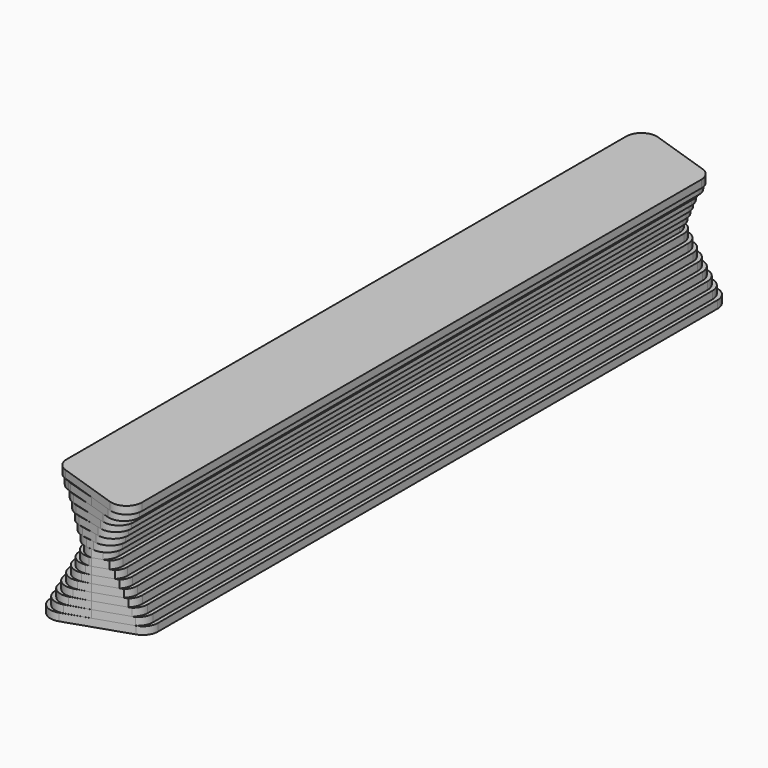
from build123d import *

# Parameters (mm, degrees)
F1_DEPTH  = 6.35
F3_DEPTH  = 6.35
F5_DEPTH  = 6.35
F7_DEPTH  = 6.35
F9_DEPTH  = 6.35
F11_DEPTH = 6.35
F13_DEPTH = 6.35
F15_DEPTH = 6.35
F17_DEPTH = 6.35
F19_DEPTH = 6.35
F21_DEPTH = 6.35
F23_DEPTH = 6.35
F25_DEPTH = 6.35
F27_DEPTH = 6.35
F29_DEPTH = 6.35
F31_DEPTH = 6.35
F33_DEPTH = 6.35


# Not quite as in the source:
# - a feature of the source that left no trace in its solid (it failed there, or was rolled back) is left out


with BuildPart() as f1:
    # F0 (on Top) → F1 (new body)
    with BuildSketch(Plane.XY):
        with BuildLine():
            Line((-38.1, 295.6463579053), (-38.1, 0))
            Line((-38.1, 0), (-38.1, -287.1796912386))
            ThreePointArc((-38.1, -287.1796912386), (-32.8258206152, -297.4824669904), (-21.3839073716, -299.2279691239))
            Line((-21.3839073716, -299.2279691239), (29.4160926284, -282.2946357905))
            ThreePointArc((29.4160926284, -282.2946357905), (35.7027757517, -277.6721785205), (38.1, -270.2463579053))
            Line((38.1, -270.2463579053), (38.1, 0))
            Line((38.1, 0), (38.1, 312.5796912386))
            ThreePointArc((38.1, 312.5796912386), (32.8258206152, 322.8824669904), (21.3839073716, 324.6279691239))
            Line((21.3839073716, 324.6279691239), (-29.4160926284, 307.6946357905))
            ThreePointArc((-29.4160926284, 307.6946357905), (-35.7027757517, 303.0721785205), (-38.1, 295.6463579053))
        make_face()
    extrude(amount=F1_DEPTH)


with BuildPart() as f3:
    # F2 (on face) → F3 (new body)
    with BuildSketch(Plane.XY.offset(6.35)):
        with BuildLine():
            Line((-34.925, 297.1010332697), (-34.925, 0))
            Line((-34.925, 0), (-34.925, -285.8442150878))
            ThreePointArc((-34.925, -285.8442150878), (-29.7212084455, -296.0958909967), (-18.3743135526, -297.946372494))
            Line((-18.3743135526, -297.946372494), (0, -292.1))
            Line((0, -292.1), (29.0322054134, -282.4225981955))
            ThreePointArc((29.0322054134, -282.4225981955), (33.3547239128, -277.8181605059), (34.925, -271.7010332697))
            Line((34.925, -271.7010332697), (34.925, 0))
            Line((34.925, 0), (34.925, 311.2442150878))
            ThreePointArc((34.925, 311.2442150878), (29.7212084455, 321.4958909967), (18.3743135526, 323.346372494))
            Line((18.3743135526, 323.346372494), (0, 317.5))
            Line((0, 317.5), (-29.0322054134, 307.8225981955))
            ThreePointArc((-29.0322054134, 307.8225981955), (-33.3547239128, 303.2181605059), (-34.925, 297.1010332697))
        make_face()
    extrude(amount=F3_DEPTH)


with BuildPart() as f5:
    # F4 (on face) → F5 (new body)
    with BuildSketch(Plane.XY.offset(12.7)):
        with BuildLine():
            Line((-31.75, 298.5258107337), (-31.75, 0))
            Line((-31.75, 0), (-31.75, -284.5558107337))
            ThreePointArc((-31.75, -284.5558107337), (-26.6310177264, -294.744930923), (-15.4006818533, -296.720204556))
            Line((-15.4006818533, -296.720204556), (0, -292.1))
            Line((0, -292.1), (26.8461437511, -283.1512854163))
            ThreePointArc((26.8461437511, -283.1512854163), (30.4583527654, -278.7060873559), (31.75, -273.1258107337))
            Line((31.75, -273.1258107337), (31.75, 0))
            Line((31.75, 0), (31.75, 309.9558107337))
            ThreePointArc((31.75, 309.9558107337), (26.6310177264, 320.144930923), (15.4006818533, 322.120204556))
            Line((15.4006818533, 322.120204556), (0, 317.5))
            Line((0, 317.5), (-26.8461437511, 308.5512854163))
            ThreePointArc((-26.8461437511, 308.5512854163), (-30.4583527654, 304.1060873559), (-31.75, 298.5258107337))
        make_face()
    extrude(amount=F5_DEPTH)


with BuildPart() as f7:
    # F6 (on face) → F7 (new body)
    with BuildSketch(Plane.XY.offset(19.05)):
        with BuildLine():
            Line((-28.575, 299.9094122505), (-28.575, 0))
            Line((-28.575, 0), (-28.575, -283.3288566949))
            ThreePointArc((-28.575, -283.3288566949), (-23.5601064147, -293.4396993598), (-12.4759229299, -295.5655341472))
            Line((-12.4759229299, -295.5655341472), (0, -292.1))
            Line((0, -292.1), (24.3225747643, -283.9924750786))
            ThreePointArc((24.3225747643, -283.9924750786), (27.4632310882, -279.7058437421), (28.575, -274.5094122505))
            Line((28.575, -274.5094122505), (28.575, 0))
            Line((28.575, 0), (28.575, 308.7288566949))
            ThreePointArc((28.575, 308.7288566949), (23.5601064147, 318.8396993598), (12.4759229299, 320.9655341472))
            Line((12.4759229299, 320.9655341472), (0, 317.5))
            Line((0, 317.5), (-24.3225747643, 309.3924750786))
            ThreePointArc((-24.3225747643, 309.3924750786), (-27.4632310882, 305.1058437421), (-28.575, 299.9094122505))
        make_face()
    extrude(amount=F7_DEPTH)


with BuildPart() as f9:
    # F8 (on face) → F9 (new body)
    with BuildSketch(Plane.XY.offset(25.4)):
        with BuildLine():
            Line((-25.4, 301.2341396387), (-25.4, 0))
            Line((-25.4, 0), (-25.4, -282.1841396387))
            ThreePointArc((-25.4, -282.1841396387), (-20.5157350594, -292.1943487015), (-9.619797562, -294.5049493905))
            Line((-9.619797562, -294.5049493905), (0, -292.1))
            Line((0, -292.1), (21.5906498503, -284.9031167166))
            ThreePointArc((21.5906498503, -284.9031167166), (24.4089976748, -280.7524089939), (25.4, -275.8341396387))
            Line((25.4, -275.8341396387), (25.4, 0))
            Line((25.4, 0), (25.4, 307.5841396387))
            ThreePointArc((25.4, 307.5841396387), (20.5157350594, 317.5943487015), (9.619797562, 319.9049493905))
            Line((9.619797562, 319.9049493905), (0, 317.5))
            Line((0, 317.5), (-21.5906498503, 310.3031167166))
            ThreePointArc((-21.5906498503, 310.3031167166), (-24.4089976748, 306.1524089939), (-25.4, 301.2341396387))
        make_face()
    extrude(amount=F9_DEPTH)


with BuildPart() as f11:
    # F10 (on face) → F11 (new body)
    with BuildSketch(Plane.XY.offset(31.75)):
        with BuildLine():
            Line((-22.225, 302.470619464), (-22.225, 0))
            Line((-22.225, 0), (-22.225, -281.1527623212))
            ThreePointArc((-22.225, -281.1527623212), (-17.509204822, -291.0291216383), (-6.8639805731, -293.57085298))
            Line((-6.8639805731, -293.57085298), (0, -292.1))
            Line((0, -292.1), (18.679051767, -285.873649411))
            ThreePointArc((18.679051767, -285.873649411), (21.3052049524, -281.8158034731), (22.225, -277.070619464))
            Line((22.225, -277.070619464), (22.225, 0))
            Line((22.225, 0), (22.225, 306.5527623212))
            ThreePointArc((22.225, 306.5527623212), (17.509204822, 316.4291216383), (6.8639805731, 318.97085298))
            Line((6.8639805731, 318.97085298), (0, 317.5))
            Line((0, 317.5), (-18.679051767, 311.273649411))
            ThreePointArc((-18.679051767, 311.273649411), (-21.3052049524, 307.2158034731), (-22.225, 302.470619464))
        make_face()
    extrude(amount=F11_DEPTH)


with BuildPart() as f13:
    # F12 (on face) → F13 (new body)
    with BuildSketch(Plane.XY.offset(38.1)):
        with BuildLine():
            Line((-19.05, 303.5664859775), (-19.05, 0))
            Line((-19.05, 0), (-19.05, -280.2831526442))
            ThreePointArc((-19.05, -280.2831526442), (-14.5589611809, -289.9735064216), (-4.2621328612, -292.8103554769))
            Line((-4.2621328612, -292.8103554769), (0, -292.1))
            Line((0, -292.1), (15.5567073259, -286.9144308914))
            ThreePointArc((15.5567073259, -286.9144308914), (18.1443881367, -282.8763064073), (19.05, -278.1664859775))
            Line((19.05, -278.1664859775), (19.05, 0))
            Line((19.05, 0), (19.05, 305.6831526442))
            ThreePointArc((19.05, 305.6831526442), (14.5589611809, 315.3735064216), (4.2621328612, 318.2103554769))
            Line((4.2621328612, 318.2103554769), (0, 317.5))
            Line((0, 317.5), (-15.5567073259, 312.3144308914))
            ThreePointArc((-15.5567073259, 312.3144308914), (-18.1443881367, 308.2763064073), (-19.05, 303.5664859775))
        make_face()
    extrude(amount=F13_DEPTH)


with BuildPart() as f15:
    # F14 (on face) → F15 (new body)
    with BuildSketch(Plane.XY.offset(44.45)):
        with BuildLine():
            Line((-15.875, 304.4191579612), (-15.875, 0))
            Line((-15.875, 0), (-15.875, -279.6541579612))
            ThreePointArc((-15.875, -279.6541579612), (-11.6967675737, -289.0706051373), (-1.9113027684, -292.2911302768))
            Line((-1.9113027684, -292.2911302768), (0, -292.1))
            Line((0, -292.1), (12.0810941165, -288.0729686278))
            ThreePointArc((12.0810941165, -288.0729686278), (14.8881847778, -283.9274471091), (15.875, -279.0191579612))
            Line((15.875, -279.0191579612), (15.875, 0))
            Line((15.875, 0), (15.875, 305.0541579612))
            ThreePointArc((15.875, 305.0541579612), (11.6967675737, 314.4706051373), (1.9113027684, 317.6911302768))
            Line((1.9113027684, 317.6911302768), (0, 317.5))
            Line((0, 317.5), (-12.0810941165, 313.4729686278))
            ThreePointArc((-12.0810941165, 313.4729686278), (-14.8881847778, 309.3274471091), (-15.875, 304.4191579612))
        make_face()
    extrude(amount=F15_DEPTH)


with BuildPart() as f17:
    # F16 (on face) → F17 (new body)
    with BuildSketch(Plane.XY.offset(50.8)):
        with BuildLine():
            Line((-12.7, 304.8), (-12.7, 0))
            Line((-12.7, 0), (-12.7, -279.4))
            ThreePointArc((-12.7, -279.4), (-8.9802561211, -288.3802561211), (0, -292.1))
            Line((0, -292.1), (7.62, -289.56))
            ThreePointArc((7.62, -289.56), (11.3592253257, -285.0796126628), (12.7, -279.4))
            Line((12.7, -279.4), (12.7, 0))
            Line((12.7, 0), (12.7, 304.8))
            ThreePointArc((12.7, 304.8), (8.9802561211, 313.7802561211), (0, 317.5))
            Line((0, 317.5), (-7.62, 314.96))
            ThreePointArc((-7.62, 314.96), (-11.3592253257, 310.4796126628), (-12.7, 304.8))
        make_face()
    extrude(amount=F17_DEPTH)


with BuildPart() as f19:
    # F18 (on face) → F19 (new body)
    with BuildSketch(Plane.XY.offset(57.15)):
        with BuildLine():
            Line((-15.875, 305.0541579612), (-15.875, 0))
            Line((-15.875, 0), (-15.875, -279.0191579612))
            ThreePointArc((-15.875, -279.0191579612), (-12.5914471761, -287.5409255348), (-4.4386972316, -291.6561302768))
            Line((-4.4386972316, -291.6561302768), (1.9113027684, -292.2911302768))
            ThreePointArc((1.9113027684, -292.2911302768), (11.6967675737, -289.0706051373), (15.875, -279.6541579612))
            Line((15.875, -279.6541579612), (15.875, 0))
            Line((15.875, 0), (15.875, 304.4191579612))
            ThreePointArc((15.875, 304.4191579612), (12.5914471761, 312.9409255348), (4.4386972316, 317.0561302768))
            Line((4.4386972316, 317.0561302768), (-1.9113027684, 317.6911302768))
            ThreePointArc((-1.9113027684, 317.6911302768), (-11.6967675737, 314.4706051373), (-15.875, 305.0541579612))
        make_face()
    extrude(amount=F19_DEPTH)


with BuildPart() as f21:
    # F20 (on face) → F21 (new body)
    with BuildSketch(Plane.XY.offset(63.5)):
        with BuildLine():
            Line((-19.05, 305.6831526442), (-19.05, 0))
            Line((-19.05, 0), (-19.05, -278.1664859775))
            ThreePointArc((-19.05, -278.1664859775), (-16.0403537774, -286.3754471584), (-8.4378671388, -290.6936888102))
            Line((-8.4378671388, -290.6936888102), (4.2621328612, -292.8103554769))
            ThreePointArc((4.2621328612, -292.8103554769), (14.5589611809, -289.9735064216), (19.05, -280.2831526442))
            Line((19.05, -280.2831526442), (19.05, 0))
            Line((19.05, 0), (19.05, 303.5664859775))
            ThreePointArc((19.05, 303.5664859775), (16.0403537774, 311.7754471584), (8.4378671388, 316.0936888102))
            Line((8.4378671388, 316.0936888102), (-4.2621328612, 318.2103554769))
            ThreePointArc((-4.2621328612, 318.2103554769), (-14.5589611809, 315.3735064216), (-19.05, 305.6831526442))
        make_face()
    extrude(amount=F21_DEPTH)


with BuildPart() as f23:
    # F22 (on face) → F23 (new body)
    with BuildSketch(Plane.XY.offset(69.85)):
        with BuildLine():
            Line((-22.225, 306.5527623212), (-22.225, 0))
            Line((-22.225, 0), (-22.225, -277.070619464))
            ThreePointArc((-22.225, -277.070619464), (-19.4013593171, -285.054824286), (-12.1860194269, -289.4887101228))
            Line((-12.1860194269, -289.4887101228), (6.8639805731, -293.57085298))
            ThreePointArc((6.8639805731, -293.57085298), (17.509204822, -291.0291216383), (22.225, -281.1527623212))
            Line((22.225, -281.1527623212), (22.225, 0))
            Line((22.225, 0), (22.225, 302.470619464))
            ThreePointArc((22.225, 302.470619464), (19.4013593171, 310.454824286), (12.1860194269, 314.8887101228))
            Line((12.1860194269, 314.8887101228), (-6.8639805731, 318.97085298))
            ThreePointArc((-6.8639805731, 318.97085298), (-17.509204822, 316.4291216383), (-22.225, 306.5527623212))
        make_face()
    extrude(amount=F23_DEPTH)


with BuildPart() as f25:
    # F24 (on face) → F25 (new body)
    with BuildSketch(Plane.XY.offset(76.2)):
        with BuildLine():
            Line((-25.4, 307.5841396387), (-25.4, 0))
            Line((-25.4, 0), (-25.4, -275.8341396387))
            ThreePointArc((-25.4, -275.8341396387), (-22.7102090628, -283.6498746981), (-15.780202438, -288.1549493905))
            Line((-15.780202438, -288.1549493905), (9.619797562, -294.5049493905))
            ThreePointArc((9.619797562, -294.5049493905), (20.5157350594, -292.1943487015), (25.4, -282.1841396387))
            Line((25.4, -282.1841396387), (25.4, 0))
            Line((25.4, 0), (25.4, 301.2341396387))
            ThreePointArc((25.4, 301.2341396387), (22.7102090628, 309.0498746981), (15.780202438, 313.5549493905))
            Line((15.780202438, 313.5549493905), (-9.619797562, 319.9049493905))
            ThreePointArc((-9.619797562, 319.9049493905), (-20.5157350594, 317.5943487015), (-25.4, 307.5841396387))
        make_face()
    extrude(amount=F25_DEPTH)


with BuildPart() as f27:
    # F26 (on face) → F27 (new body)
    with BuildSketch(Plane.XY.offset(82.55)):
        with BuildLine():
            Line((-28.575, 308.7288566949), (-28.575, 0))
            Line((-28.575, 0), (-28.575, -274.5094122505))
            ThreePointArc((-28.575, -274.5094122505), (-25.9858426649, -282.1945186651), (-19.2740770701, -286.7460897028))
            Line((-19.2740770701, -286.7460897028), (12.4759229299, -295.5655341472))
            ThreePointArc((12.4759229299, -295.5655341472), (23.5601064147, -293.4396993598), (28.575, -283.3288566949))
            Line((28.575, -283.3288566949), (28.575, 0))
            Line((28.575, 0), (28.575, 299.9094122505))
            ThreePointArc((28.575, 299.9094122505), (25.9858426649, 307.5945186651), (19.2740770701, 312.1460897028))
            Line((19.2740770701, 312.1460897028), (-12.4759229299, 320.9655341472))
            ThreePointArc((-12.4759229299, 320.9655341472), (-23.5601064147, 318.8396993598), (-28.575, 308.7288566949))
        make_face()
    extrude(amount=F27_DEPTH)


with BuildPart() as f29:
    # F28 (on face) → F29 (new body)
    with BuildSketch(Plane.XY.offset(88.9)):
        with BuildLine():
            Line((-31.75, 309.9558107337), (-31.75, 0))
            Line((-31.75, 0), (-31.75, -273.1258107337))
            ThreePointArc((-31.75, -273.1258107337), (-29.2391201893, -280.7068284601), (-22.6993181467, -285.290204556))
            Line((-22.6993181467, -285.290204556), (15.4006818533, -296.720204556))
            ThreePointArc((15.4006818533, -296.720204556), (26.6310177264, -294.744930923), (31.75, -284.5558107337))
            Line((31.75, -284.5558107337), (31.75, 0))
            Line((31.75, 0), (31.75, 298.5258107337))
            ThreePointArc((31.75, 298.5258107337), (29.2391201893, 306.1068284601), (22.6993181467, 310.690204556))
            Line((22.6993181467, 310.690204556), (-15.4006818533, 322.120204556))
            ThreePointArc((-15.4006818533, 322.120204556), (-26.6310177264, 320.144930923), (-31.75, 309.9558107337))
        make_face()
    extrude(amount=F29_DEPTH)


with BuildPart() as f31:
    # F30 (on face) → F31 (new body)
    with BuildSketch(Plane.XY.offset(88.9)):
        with BuildLine():
            Line((-34.925, 311.2442150878), (-34.925, 0))
            Line((-34.925, 0), (-34.925, -271.7010332697))
            ThreePointArc((-34.925, -271.7010332697), (-32.4766759089, -279.1972417152), (-26.0756864474, -283.8031906758))
            Line((-26.0756864474, -283.8031906758), (18.3743135526, -297.946372494))
            ThreePointArc((18.3743135526, -297.946372494), (29.7212084455, -296.0958909967), (34.925, -285.8442150878))
            Line((34.925, -285.8442150878), (34.925, 0))
            Line((34.925, 0), (34.925, 297.1010332697))
            ThreePointArc((34.925, 297.1010332697), (32.4766759089, 304.5972417152), (26.0756864474, 309.2031906758))
            Line((26.0756864474, 309.2031906758), (-18.3743135526, 323.346372494))
            ThreePointArc((-18.3743135526, 323.346372494), (-29.7212084455, 321.4958909967), (-34.925, 311.2442150878))
        make_face()
    extrude(amount=F31_DEPTH)


with BuildPart() as f33:
    # F32 (on face) → F33 (new body)
    with BuildSketch(Plane.XY.offset(95.25)):
        with BuildLine():
            Line((-38.1, 312.5796912386), (-38.1, 0))
            Line((-38.1, 0), (-38.1, -270.2463579053))
            ThreePointArc((-38.1, -270.2463579053), (-35.7027757517, -277.6721785205), (-29.4160926284, -282.2946357905))
            Line((-29.4160926284, -282.2946357905), (21.3839073716, -299.2279691239))
            ThreePointArc((21.3839073716, -299.2279691239), (32.8258206152, -297.4824669904), (38.1, -287.1796912386))
            Line((38.1, -287.1796912386), (38.1, 0))
            Line((38.1, 0), (38.1, 295.6463579053))
            ThreePointArc((38.1, 295.6463579053), (35.7027757517, 303.0721785205), (29.4160926284, 307.6946357905))
            Line((29.4160926284, 307.6946357905), (-21.3839073716, 324.6279691239))
            ThreePointArc((-21.3839073716, 324.6279691239), (-32.8258206152, 322.8824669904), (-38.1, 312.5796912386))
        make_face()
    extrude(amount=F33_DEPTH)


solid = Compound([f1.part, f3.part, f5.part, f7.part, f9.part, f11.part, f13.part, f15.part, f17.part, f19.part, f21.part, f23.part, f25.part, f27.part, f29.part, f31.part, f33.part])
